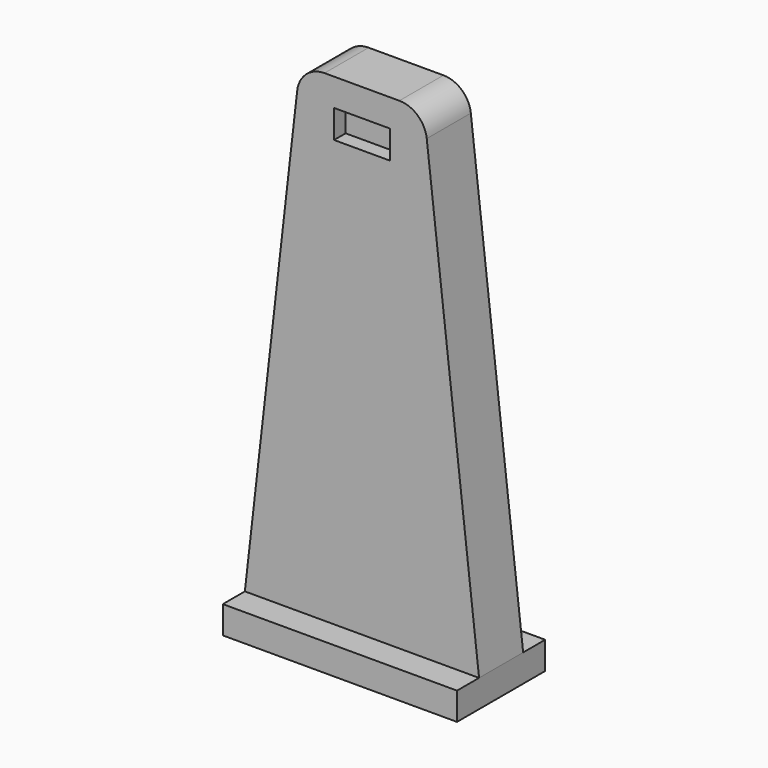
from build123d import *

# Parameters (mm, degrees)
F0_W          = 9
F0_H          = 4
F2_W          = 17
F2_H          = 4
F4_DEPTH      = 2
F5_W          = 17
F5_H          = 2
F6_DEPTH      = 2
F6_DEPTH_BACK = 6
F7_W          = 4.05
F7_H          = 2.05
F8_DEPTH      = 1.05
F9_W          = 14.9999996647
F9_H          = 5.9999996647
F10_DEPTH     = 1
F11_R         = 2


with BuildPart() as f3:
    # F0 (on Top) → F3 section 0
    with BuildSketch(Plane.XY):
        Rectangle(F0_W, F0_H)
    # F2 (on offset) → F3 section 1
    with BuildSketch(Plane.XY.offset(-35)):
        Rectangle(F2_W, F2_H)
    loft()

    # F4 (add): a face of the model
    f4_faces = [f3.faces().sort_by_distance(p)[0] for p in [
        (0, 0, -35),
    ]]
    extrude(f4_faces, amount=F4_DEPTH)

    # F5 (on face) → F6 (join, two sides)
    with BuildSketch(Plane.XZ.offset(2)) as f6_sk:
        with Locations((0, -36)):
            Rectangle(F5_W, F5_H)
    extrude(amount=F6_DEPTH)
    extrude(f6_sk.sketch, amount=-F6_DEPTH_BACK)

    # F7 (on face) → F8 (cut)
    with BuildSketch(Plane.XZ.offset(2)):
        with Locations((0, -3.025)):
            Rectangle(F7_W, F7_H)
    extrude(amount=-F8_DEPTH, mode=Mode.SUBTRACT)

    # F9 (on face) → F10 (cut)
    with BuildSketch(Plane(origin=(0, 0, -37), x_dir=(1, 0, 0), z_dir=(0, 0, -1))):
        Rectangle(F9_W, F9_H)
    extrude(amount=-F10_DEPTH, mode=Mode.SUBTRACT)

    # F11
    f11_edges = [f3.edges().sort_by_distance(p)[0] for p in [
        (-4.5, 0, 0),
        (4.5, 0, 0),
    ]]
    fillet(f11_edges, radius=F11_R)


solid = f3.part
